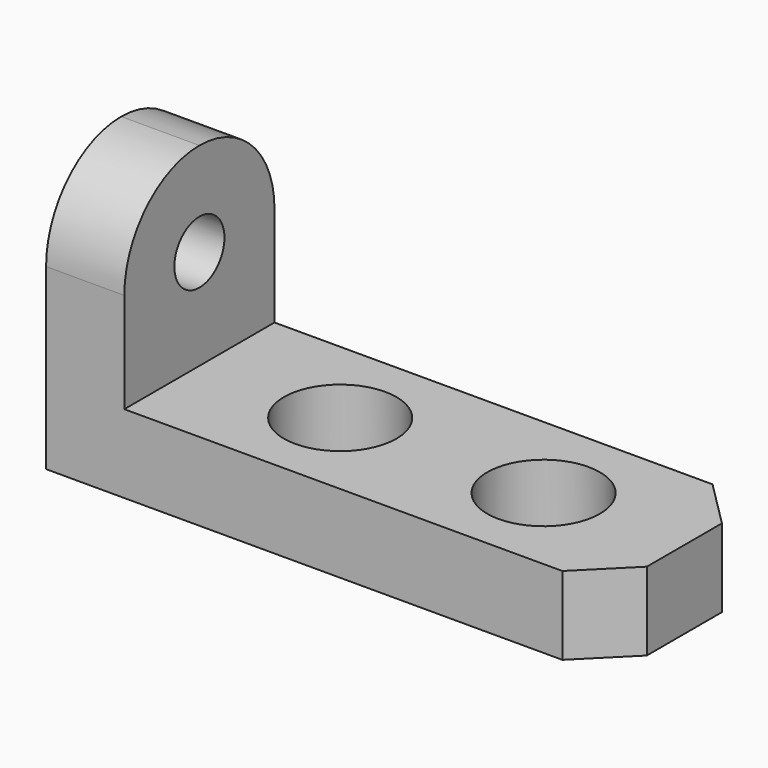
from build123d import *

# Parameters (mm, degrees)
F0_W      = 180
F0_H      = 60
F1_DEPTH  = 25
F2_W      = 25
F2_H      = 60
F3_DEPTH  = 62
F4_R      = 30
F5_R      = 29.99999
F6_R      = 18
F7_DEPTH  = 25
F8_SIZE   = 15
F9_R      = 10
F10_DEPTH = 25.001


# Not quite as in the source:
# - a fillet or chamfer is up to 0.001 mm smaller than in the source, because OpenCascade refuses the exact size


with BuildPart() as f1:
    # F0 (on Top) → F1 (new body)
    with BuildSketch(Plane.XY):
        with Locations((90, 30)):
            Rectangle(F0_W, F0_H)
    extrude(amount=F1_DEPTH)

    # F2 (on face) → F3 (join)
    with BuildSketch(Plane.XY.offset(25)):
        with Locations((12.5, 30)):
            Rectangle(F2_W, F2_H)
    extrude(amount=F3_DEPTH)

    # F4
    f4_edges = [f1.edges().sort_by_distance(p)[0] for p in [
        (12.5, 0, 87),
    ]]
    fillet(f4_edges, radius=F4_R)

    # F5 (radius 30 in the source; OpenCascade refuses exactly that, so slightly less here)
    f5_edges = [f1.edges().sort_by_distance(p)[0] for p in [
        (12.5, 60, 87),
    ]]
    fillet(f5_edges, radius=F5_R)

    # F6 (on face) → F7 (cut)
    with BuildSketch(Plane.XY.offset(25)):
        with Locations((70, 30)):
            Circle(F6_R)
        with Locations((135, 30)):
            Circle(F6_R)
    extrude(amount=-F7_DEPTH, mode=Mode.SUBTRACT)

    # F8
    f8_edges = [f1.edges().sort_by_distance(p)[0] for p in [
        (180, 0, 12.5),
        (180, 60, 12.5),
    ]]
    chamfer(f8_edges, length=F8_SIZE)

    # F9 (on face) → F10 (cut, through all)
    with BuildSketch(Plane.YZ.offset(25)):
        with Locations((30, 57)):
            Circle(F9_R)
    extrude(amount=-F10_DEPTH, mode=Mode.SUBTRACT)


solid = f1.part
